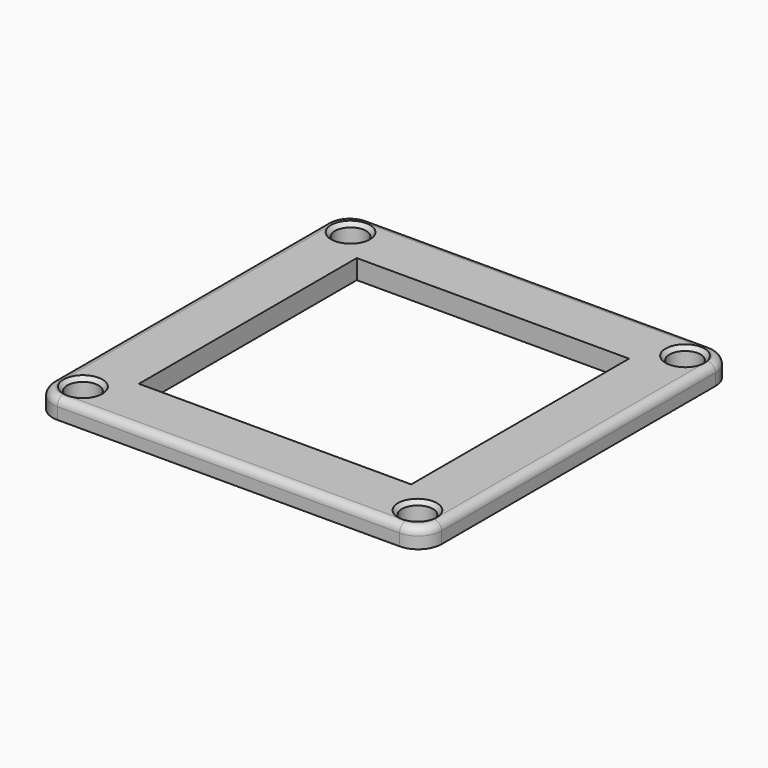
from build123d import *

# Parameters (mm, degrees)
F0_W     = 50
F0_H     = 50
F0_R     = 2
F0_W_2   = 35
F0_H_2   = 35
F1_DEPTH = 2.5
F2_R     = 3
F3_SIZE  = 0.5
F4_R     = 0.99999


# Not quite as in the source:
# - a fillet or chamfer is up to 0.001 mm smaller than in the source, because OpenCascade refuses the exact size


with BuildPart() as f1:
    # F0 (on Top) → F1 (new body)
    with BuildSketch(Plane.XY):
        with Locations((11.1718769372, 3.8648895919)):
            Rectangle(F0_W, F0_H)
        with Locations((-10.3281230628, -17.6351104081)):
            Circle(F0_R, mode=Mode.SUBTRACT)
        with Locations((32.6718769372, -17.6351104081)):
            Circle(F0_R, mode=Mode.SUBTRACT)
        with Locations((11.1718769372, 3.8648895919)):
            Rectangle(F0_W_2, F0_H_2, mode=Mode.SUBTRACT)
        with Locations((-10.3281230628, 25.3648895919)):
            Circle(F0_R, mode=Mode.SUBTRACT)
        with Locations((32.6718769372, 25.3648895919)):
            Circle(F0_R, mode=Mode.SUBTRACT)
    extrude(amount=F1_DEPTH)

    # F2
    f2_edges = [f1.edges().sort_by_distance(p)[0] for p in [
        (-13.828123, 28.86489, 1.25),
        (36.171877, 28.86489, 1.25),
        (36.171877, -21.13511, 1.25),
        (-13.828123, -21.13511, 1.25),
    ]]
    fillet(f2_edges, radius=F2_R)

    # F3
    f3_edges = [f1.edges().sort_by_distance(p)[0] for p in [
        (-12.328123, 25.36489, 2.5),
        (30.671877, 25.36489, 2.5),
        (30.671877, -17.63511, 2.5),
        (-12.328123, -17.63511, 2.5),
    ]]
    chamfer(f3_edges, length=F3_SIZE)

    # F4 (radius 1 in the source; OpenCascade refuses exactly that, so slightly less here)
    f4_edges = [f1.edges().sort_by_distance(p)[0] for p in [
        (11.171877, 28.86489, 2.5),
    ]]
    fillet(f4_edges, radius=F4_R)


solid = f1.part
